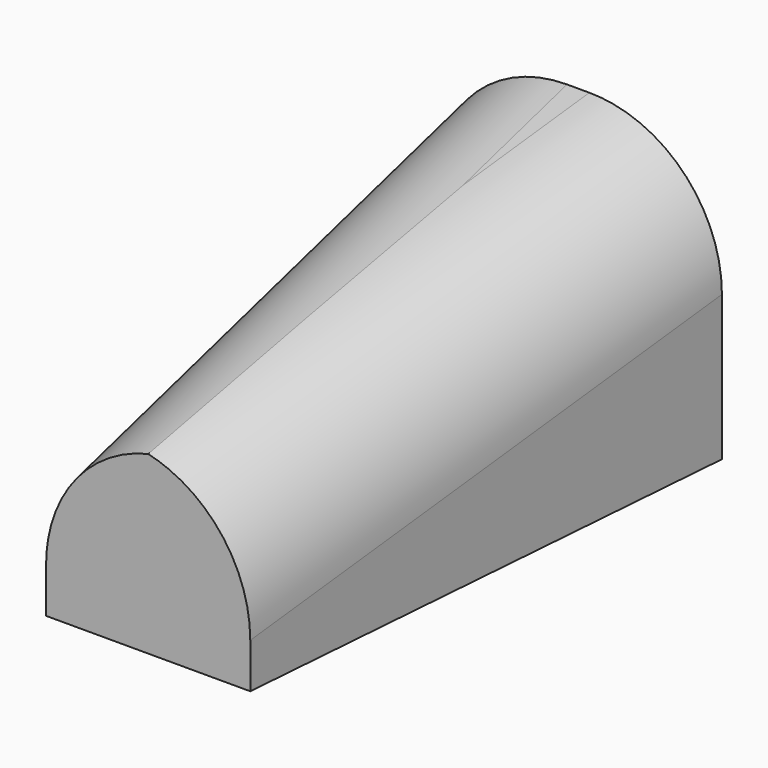
from build123d import *

# Parameters (mm, degrees)
F0_W        = 54.4569883496
F0_H        = 52.9484525323
F2_W        = 38.669379428
F2_H        = 33.9629091322
F4_T1_DEPTH = 228.8872093308
F4_T3_DEPTH = 228.8436040844


# Not quite as in the source:
# - a fillet or chamfer that OpenCascade refuses, or shapes differently, is made with other operations: its cross-section is extruded or revolved along the edge and cut away or added


with BuildPart() as f3:
    # F0 (on Front) → F3 section 0
    with BuildSketch(Plane.XZ):
        with Locations((-0.4889173433, 26.4742262661)):
            Rectangle(F0_W, F0_H)
    # F2 (on offset) → F3 section 1
    with BuildSketch(Plane.XZ.offset(101.6)):
        with Locations((-0.6360104308, 16.9814545661)):
            Rectangle(F2_W, F2_H)
    loft()

    # F4: fillet of radius 25.4 on 2 edges, made by hand

    # F4_s2 → F4_t1 (cut)
    with BuildSketch(Plane(origin=(-5.5598937152, 72.9193556138, 13.6261180188), x_dir=(0.9971057986, 0.0760264846, 0), z_dir=(0.0747401792, -0.9802355917, -0.1831722969))):
        with BuildLine():
            ThreePointArc((-2.5919028833, 52.0164089613), (-20.3226785097, 44.4535478513), (-27.6371917475, 26.6188858536))
            Line((-27.6371917475, 26.6188858536), (-27.6371917475, 51.6666172583))
            Line((-27.6371917475, 51.6666172583), (-2.5919028833, 52.0164089613))
        make_face()
    extrude(amount=F4_T1_DEPTH, mode=Mode.SUBTRACT)

    # F4_s4 → F4_t3 (cut)
    with BuildSketch(Plane(origin=(5.7672479515, 72.8715156932, 13.6171783841), x_dir=(0.9968828528, -0.078895993, 0), z_dir=(-0.0775617197, -0.9800237693, -0.1831327146))):
        with BuildLine():
            ThreePointArc((1.6243248242, 52.0294565484), (19.3464124697, 44.4620185205), (26.6562256355, 26.6321239525))
            Line((26.6562256355, 26.6321239525), (26.6562256355, 51.6666537877))
            Line((26.6562256355, 51.6666537877), (1.6243248242, 52.0294565484))
        make_face()
    extrude(amount=F4_T3_DEPTH, mode=Mode.SUBTRACT)


solid = f3.part
